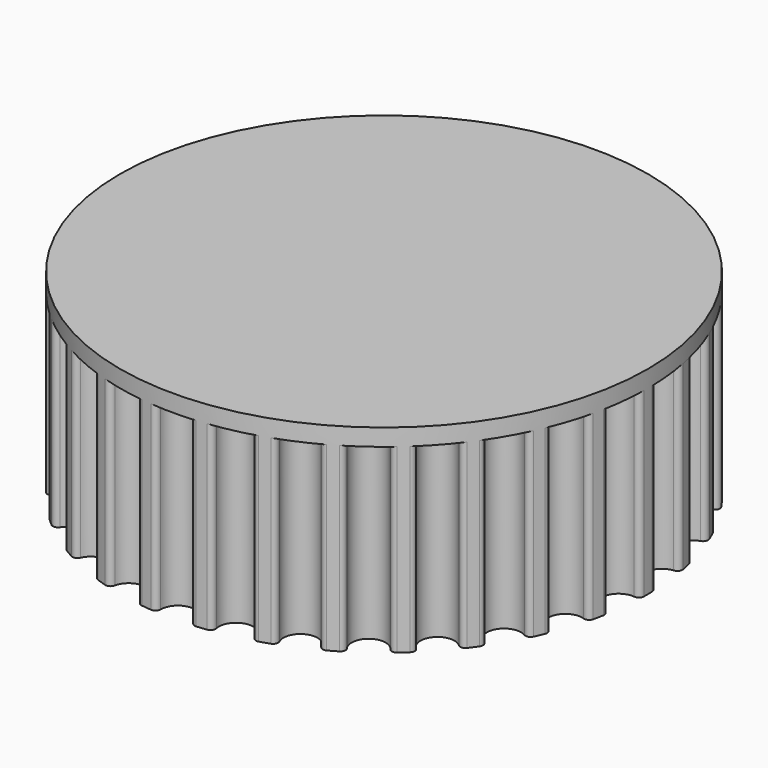
from build123d import *

# Parameters (mm, degrees)
F2_R            = 23.3007414911
F3_DEPTH        = 16
F5_DEPTH        = 16
F5_COPIES_COUNT = 30
F7_R            = 23.3007414911
F8_DEPTH        = 1.5


# Not quite as in the source:
# - a feature of the source that left no trace in its solid (it failed there, or was rolled back) is left out
# - a pattern or mirror of a feature is missing from the dataset's text; its kind, count and spacing are read off the source's solid


with BuildPart() as f3:
    # F2 (on Top) → F3 (new body)
    with BuildSketch(Plane.XY):
        Circle(F2_R)
    extrude(amount=F3_DEPTH)

    # F4 (on face) → F5 (cut, through all)
    with BuildSketch(Plane.XY.offset(16)):
        with BuildLine():
            ThreePointArc((-1.9882155288, 23.2157608758), (-1.6432389463, 23.0968097974), (-1.4998597988, 22.7612496365))
            ThreePointArc((-1.4998597988, 22.7612496365), (0, 21.2407414911), (1.4998597988, 22.7612496365))
            ThreePointArc((1.4998597988, 22.7612496365), (1.6432389463, 23.0968097974), (1.9882155288, 23.2157608758))
            ThreePointArc((1.9882155288, 23.2157608758), (0, 23.3007414911), (-1.9882155288, 23.2157608758))
        make_face()
    f5 = extrude(amount=-F5_DEPTH, mode=Mode.SUBTRACT)

    # F5_copies: F5 ×30 about axis
    f5_copies_axis = Axis((0, 0, 0), (0, 0, 1))
    for i in range(1, F5_COPIES_COUNT):
        add(f5.rotate(f5_copies_axis, i * 360 / F5_COPIES_COUNT), mode=Mode.SUBTRACT)

    # F7 (on face) → F8 (join)
    with BuildSketch(Plane.XY.offset(16)):
        Circle(F7_R)
    extrude(amount=F8_DEPTH)


solid = f3.part
